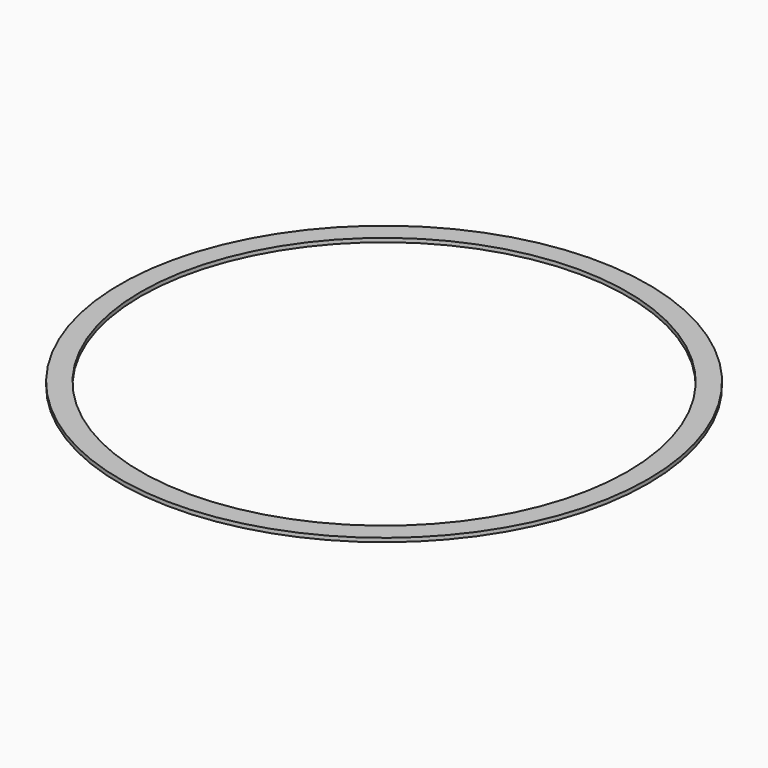
from build123d import *

# Parameters (mm, degrees)
F0_R     = 325.54926
F0_R_2   = 300.14926
F1_DEPTH = 4.7625


# Not quite as in the source:
# - a length typed as a fraction of an inch, garbled in the dataset ("3 / 203.2 mm" for 3/8 in), is restored


with BuildPart() as f1:
    # F0 (on Top) → F1 (new body)
    with BuildSketch(Plane.XY):
        Circle(F0_R)
        Circle(F0_R_2, mode=Mode.SUBTRACT)
    extrude(amount=F1_DEPTH)


solid = f1.part
